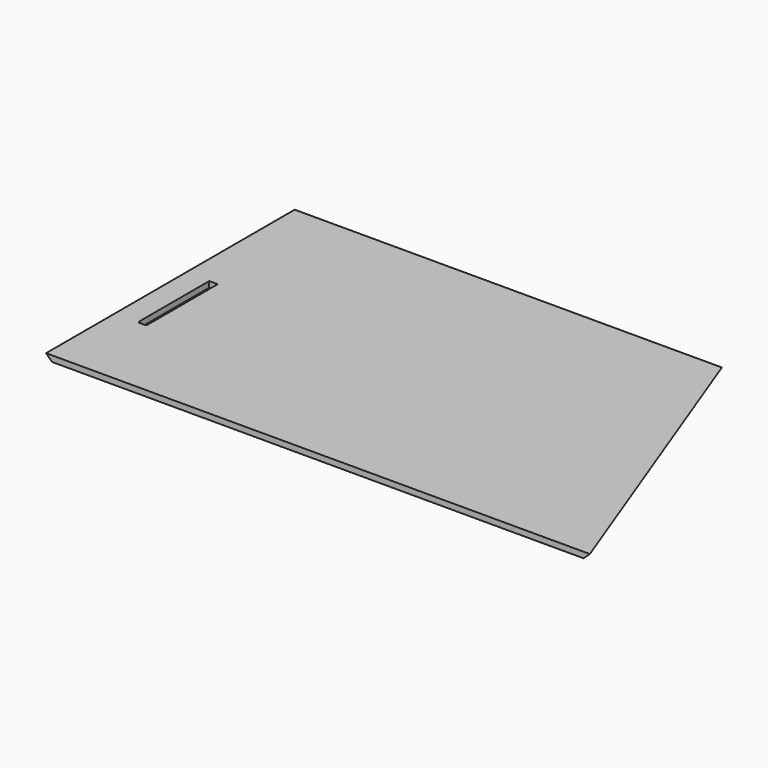
from build123d import *

# Parameters (mm, degrees)
F1_DEPTH = 15
F2_SIZE  = 14.99999
F3_SIZE  = 14.99999


# Not quite as in the source:
# - a fillet or chamfer is up to 0.001 mm smaller than in the source, because OpenCascade refuses the exact size


with BuildPart() as f1:
    # F0 (on Top) → F1 (new body)
    with BuildSketch(Plane.XY):
        Polygon((0, -800), (-300, 0), (-1400, 0), (-1400, -800), align=None)
        with BuildLine():
            Line((-1340, -575), (-1340, -350))
            Line((-1340, -350), (-1318, -350))
            Line((-1318, -350), (-1318, -575))
            ThreePointArc((-1318, -575), (-1319.4644660941, -578.5355339059), (-1323, -580))
            Line((-1323, -580), (-1335, -580))
            ThreePointArc((-1335, -580), (-1338.5355339059, -578.5355339059), (-1340, -575))
        make_face(mode=Mode.SUBTRACT)
    extrude(amount=F1_DEPTH)

    # F2 (size 15 in the source; OpenCascade refuses exactly that, so slightly less here)
    f2_edges = [f1.edges().sort_by_distance(p)[0] for p in [
        (-1400, -400, 0),
    ]]
    chamfer(f2_edges, length=F2_SIZE)

    # F3 (size 15 in the source; OpenCascade refuses exactly that, so slightly less here)
    f3_edges = [f1.edges().sort_by_distance(p)[0] for p in [
        (-150, -400, 0),
    ]]
    chamfer(f3_edges, length=F3_SIZE)


solid = f1.part
